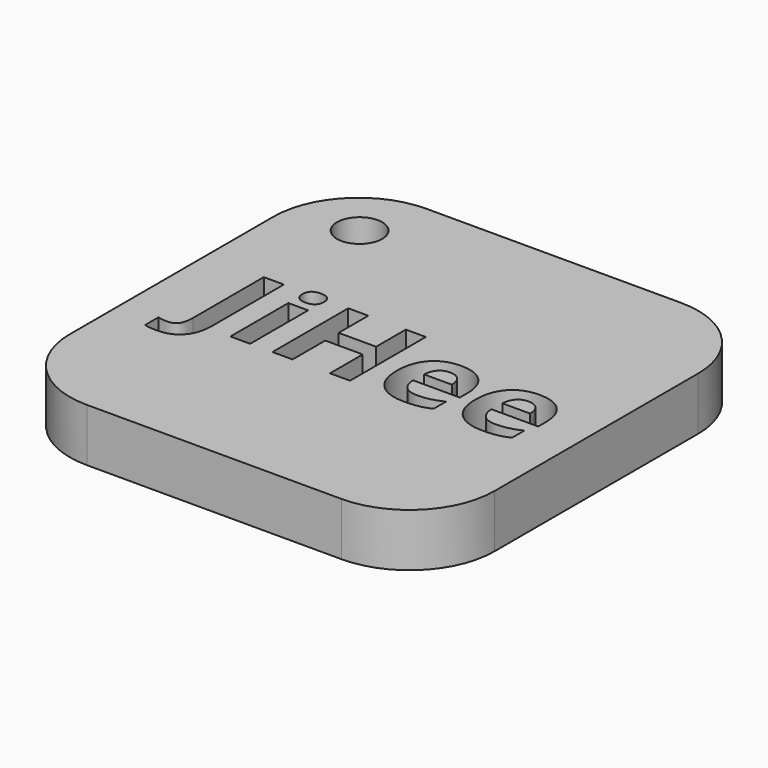
from build123d import *

# Parameters (mm, degrees)
F1_DEPTH     = 5
F2_R         = 2.1317877857
F2_TEXT_SIZE = 12.5
F3_DEPTH     = 10


# Not quite as in the source:
# - Text() gives the source's letters only with a copy of the font that has no kerning and outlines rounded to 1/6400 em; it was checked with that copy


with BuildPart() as f1:
    # F0 (on Top) → F1 (new body)
    with BuildSketch(Plane.XY):
        with BuildLine():
            ThreePointArc((20, 12), (17.6568542495, 17.6568542495), (12, 20))
            Line((12, 20), (-12, 20))
            ThreePointArc((-12, 20), (-17.6568542495, 17.6568542495), (-20, 12))
            Line((-20, 12), (-20, -12))
            ThreePointArc((-20, -12), (-17.6568542495, -17.6568542495), (-12, -20))
            Line((-12, -20), (12, -20))
            ThreePointArc((12, -20), (17.6568542495, -17.6568542495), (20, -12))
            Line((20, -12), (20, 12))
        make_face()
    extrude(amount=F1_DEPTH)

    # F2 (on face) → F3 (cut)
    with BuildSketch(Plane.XY.offset(5)):
        with Locations((-13.6698884889, 14.2152346671)):
            Circle(F2_R)
        with Locations((-15.6661194793, -4.9004718862)):
            Text('JiHee', F2_TEXT_SIZE, font='Open Sans', font_style=FontStyle.BOLD, text_align=(TextAlign.LEFT, TextAlign.BOTTOM))
    extrude(amount=-F3_DEPTH, mode=Mode.SUBTRACT)


solid = f1.part
